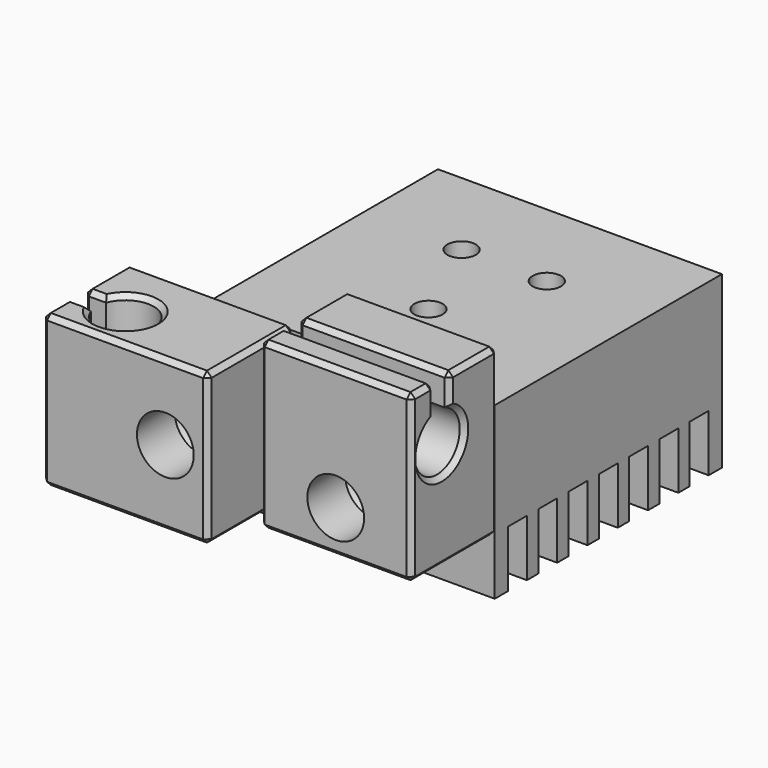
from build123d import *

# Parameters (mm, degrees)
F0_W            = 30
F0_H            = 30
F11_DEPTH       = 18
F1_D            = 5
F1_DEPTH        = 20
F1_TIP          = 1.5021515476
F13_W           = 30
F13_H           = 2.5
F14_DEPTH       = 6
F15_D           = 3
F15_DEPTH       = 3
F15_TIP         = 0.9012909285
F16_D           = 3
F16_DEPTH       = 10
F16_TIP         = 0.9012909285
F3_R            = 1.475
F4_DEPTH        = 2.1
F18_W           = 17.5
F18_H           = 16
F17_W           = 16
F17_H           = 17.5
F19_DEPTH       = 11.4
F5_D            = 6
F5_DEPTH        = 5
F5_TIP          = 1.8025818571
F5_ON_F20_D     = 6
F5_ON_F20_DEPTH = 5
F5_ON_F20_TIP   = 1.8025818571
F8_DEPTH        = 16
F7_W            = 1.3441740274
F7_H            = 2
F22_DEPTH       = 16
F9_SIZE         = 0.49999


# Not quite as in the source:
# - a fillet or chamfer is up to 0.001 mm smaller than in the source, because OpenCascade refuses the exact size


with BuildPart() as f11:
    # F0 (on Top) → F11 (new body)
    with BuildSketch(Plane.XY):
        Rectangle(F0_W, F0_H)
    extrude(amount=F11_DEPTH)

    # F1
    with Locations(Plane(origin=(0, 15, 0), x_dir=(-1, 0, 0), z_dir=(0, 1, 0))):
        with Locations((-9, 12), (9, 12)):
            Hole(F1_D / 2, depth=F1_DEPTH)
            with Locations((0, 0, -(F1_DEPTH + F1_TIP / 2))):  # 118° drill point
                Cone(0, F1_D / 2, F1_TIP, mode=Mode.SUBTRACT)

    # F13 (on face) → F14 (cut)
    with BuildSketch(Plane(origin=(0, 0, 0), x_dir=(1, 0, 0), z_dir=(0, 0, -1))):
        with Locations((0, 12)):
            Rectangle(F13_W, F13_H)
        with Locations((0, 8)):
            Rectangle(F13_W, F13_H)
        with Locations((0, 4)):
            Rectangle(F13_W, F13_H)
        Rectangle(F13_W, F13_H)
        with Locations((0, -4)):
            Rectangle(F13_W, F13_H)
        with Locations((0, -8)):
            Rectangle(F13_W, F13_H)
        with Locations((0, -12)):
            Rectangle(F13_W, F13_H)
    extrude(amount=-F14_DEPTH, mode=Mode.SUBTRACT)

    # F15
    with Locations(Plane.XY.offset(18)):
        with Locations((4.5, 5), (-4.5, 5), (0, -5)):
            Hole(F15_D / 2, depth=F15_DEPTH)
            with Locations((0, 0, -(F15_DEPTH + F15_TIP / 2))):  # 118° drill point
                Cone(0, F15_D / 2, F15_TIP, mode=Mode.SUBTRACT)

    # F16
    with Locations(Plane(origin=(0, 15, 0), x_dir=(-1, 0, 0), z_dir=(0, 1, 0))):
        with Locations((8.5, 3), (-8.5, 3), (0, 15)):
            Hole(F16_D / 2, depth=F16_DEPTH)
            with Locations((0, 0, -(F16_DEPTH + F16_TIP / 2))):  # 118° drill point
                Cone(0, F16_D / 2, F16_TIP, mode=Mode.SUBTRACT)

    # F3 (on face) → F4 (join)
    with BuildSketch(Plane.XZ.offset(15)):
        with Locations((-9, 12)):
            Circle(F3_R)
        with Locations((9, 12)):
            Circle(F3_R)
    extrude(amount=F4_DEPTH)

    # F18 (on face) + F17 (on face) → F19 (join)
    with BuildSketch(Plane.XZ.offset(17.1)):
        with Locations((-13.25, 12)):
            Rectangle(F18_W, F18_H)
    with BuildSketch(Plane.XZ.offset(17.1)):
        with Locations((9, 16.25)):
            Rectangle(F17_W, F17_H)
    extrude(amount=F19_DEPTH)

    # F5
    with Locations(Plane.XZ.offset(28.5)):
        with Locations((-9, 12)):
            Hole(F5_D / 2, depth=F5_DEPTH)
            with Locations((0, 0, -(F5_DEPTH + F5_TIP / 2))):  # 118° drill point
                Cone(0, F5_D / 2, F5_TIP, mode=Mode.SUBTRACT)

    # F5 on F20
    with Locations(Plane.XZ.offset(28.5)):
        with Locations((9, 12)):
            Hole(F5_ON_F20_D / 2, depth=F5_ON_F20_DEPTH)
            with Locations((0, 0, -(F5_ON_F20_DEPTH + F5_ON_F20_TIP / 2))):  # 118° drill point
                Cone(0, F5_ON_F20_D / 2, F5_ON_F20_TIP, mode=Mode.SUBTRACT)

    # F6 (on face) → F8 (cut, through all)
    with BuildSketch(Plane.YZ.offset(17)):
        with BuildLine():
            Line((-25.5, 25), (-25.5, 21.7284271247))
            ThreePointArc((-25.5, 21.7284271247), (-24.5, 15.9), (-23.5, 21.7284271247))
            Line((-23.5, 21.7284271247), (-23.5, 25))
            Line((-23.5, 25), (-25.5, 25))
        make_face()
    extrude(amount=-F8_DEPTH, mode=Mode.SUBTRACT)

    # F7 (on face) → F22 (cut, through all)
    with BuildSketch(Plane.XY.offset(20)):
        with BuildLine():
            Line((-22, -24.9799899757), (-19.6726011522, -24.9799899757))
            ThreePointArc((-19.6726011522, -24.9799899757), (-16.8441740274, -26.9799899757), (-14.0157469027, -24.9799899757))
            ThreePointArc((-14.0157469027, -24.9799899757), (-15.8441740274, -21.1515628509), (-19.6726011522, -22.9799899757))
            Line((-19.6726011522, -22.9799899757), (-22, -22.9799899757))
            Line((-22, -22.9799899757), (-22, -24.9799899757))
        make_face()
        with Locations((-22.6720870137, -23.9799899757)):
            Rectangle(F7_W, F7_H)
    extrude(amount=-F22_DEPTH, mode=Mode.SUBTRACT)

    # F9 (size 0.5 in the source; OpenCascade refuses exactly that, so slightly less here)
    f9_edges = [f11.edges().sort_by_distance(p)[0] for p in [
        (17, -17.1, 16.25),
        (17, -20.3, 25),
        (17, -23.5, 23.364214),
        (17, -24.5, 15.9),
        (17, -25.5, 23.364214),
        (17, -27, 25),
        (17, -28.5, 16.25),
        (17, -22.8, 7.5),
        (1, -22.8, 7.5),
        (9, -17.1, 7.5),
        (9, -28.5, 7.5),
        (-13.25, -17.1, 4),
        (-4.5, -22.8, 4),
        (-13.25, -28.5, 4),
        (-22, -26.739995, 4),
        (-20.836301, -24.97999, 4),
        (-13.844174, -23.97999, 4),
        (-20.836301, -22.97999, 4),
        (-22, -20.039995, 4),
        (-4.5, -22.8, 20),
        (-4.5, -17.1, 12),
        (-4.5, -28.5, 12),
        (9, -17.1, 25),
        (1, -20.3, 25),
        (9, -23.5, 25),
        (9, -25.5, 25),
        (1, -27, 25),
        (9, -28.5, 25),
        (-13.25, -17.1, 20),
        (-22, -20.039995, 20),
        (-20.836301, -22.97999, 20),
        (-13.844174, -23.97999, 20),
        (-20.836301, -24.97999, 20),
        (-22, -26.739995, 20),
        (-13.25, -28.5, 20),
        (-22, -17.1, 12),
        (-22, -22.97999, 12),
        (1, -17.1, 16.25),
        (1, -28.5, 16.25),
        (1, -25.5, 23.364214),
        (1, -24.5, 15.9),
        (1, -23.5, 23.364214),
        (-22, -24.97999, 12),
        (-22, -28.5, 12),
    ]]
    chamfer(f9_edges, length=F9_SIZE)


solid = f11.part
